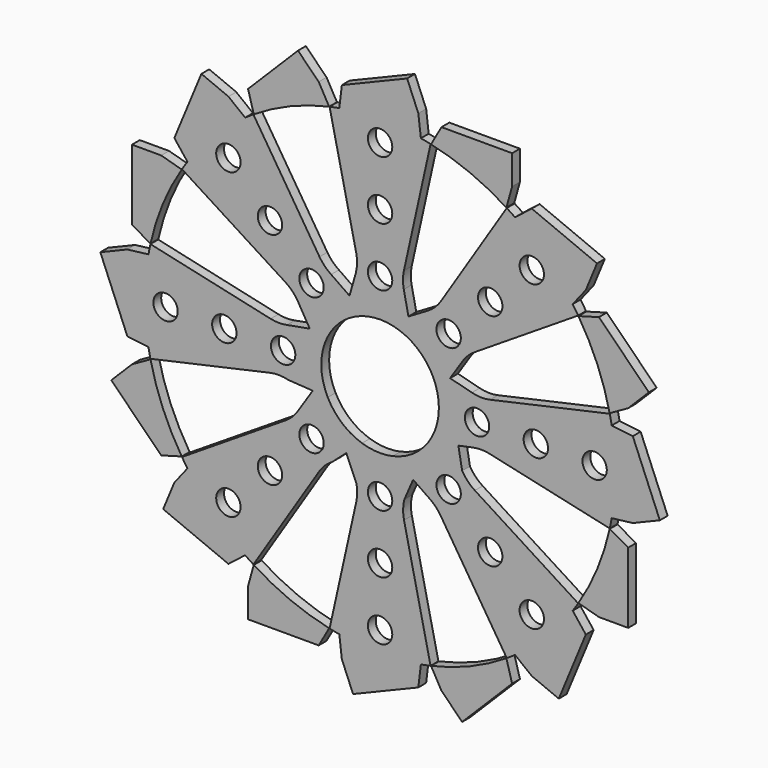
from build123d import *

# Parameters (mm, degrees)
F0_R     = 3.9501817168
F1_DEPTH = 3.175


# Not quite as in the source:
# - a feature names something its author has since deleted; it is built from what else it names


with BuildPart() as f1:
    # F0 (on Front) → F1 (new body)
    with BuildSketch(Plane.XZ):
        with BuildLine():
            ThreePointArc((-16.0654565205, 10.2373632733), (-10.9248771439, 15.6060744388), (-4.1210842565, 18.5989022405))
            Line((-4.1210842565, 18.5989022405), (-9.8997067311, 22.600704596))
            Line((-9.8997067311, 22.600704596), (-15.8721102734, 26.7367039053))
            ThreePointArc((-15.8721102734, 26.7367039053), (-17.9521481778, 28.4386641703), (-19.6274585749, 30.5402258516))
            Line((-19.6274585749, 30.5402258516), (-41.056319087, 64.1936029759))
            ThreePointArc((-41.056319087, 64.1936029759), (-42.3978695177, 63.3155641242), (-43.7206489599, 62.4094933045))
            ThreePointArc((-43.7206489599, 62.4094933045), (-53.8815367264, 53.8815367264), (-62.4094933045, 43.7206489599))
            ThreePointArc((-62.4094933045, 43.7206489599), (-63.3155641242, 42.3978695177), (-64.1936029759, 41.056319087))
            Line((-64.1936029759, 41.056319087), (-30.7105790862, 19.7359313647))
            ThreePointArc((-30.7105790862, 19.7359313647), (-28.3975370068, 17.8468155599), (-26.5895994967, 15.4697829255))
            Line((-26.5895994967, 15.4697829255), (-22.7875423577, 9.0161548324))
            Line((-22.7875423577, 9.0161548324), (-16.0654565205, 10.2373632733))
        make_face()
        with Locations((-22.2146216346, 22.2146216346)):
            Circle(F0_R, mode=Mode.SUBTRACT)
        with Locations((-35.6850058163, 35.6850058163)):
            Circle(F0_R, mode=Mode.SUBTRACT)
        with Locations((-49.1553899979, 49.1553899979)):
            Circle(F0_R, mode=Mode.SUBTRACT)
        with BuildLine():
            Line((30.5402258516, 19.6274585749), (64.1936029759, 41.056319087))
            ThreePointArc((64.1936029759, 41.056319087), (63.3155641242, 42.3978695177), (62.4094933045, 43.7206489599))
            ThreePointArc((62.4094933045, 43.7206489599), (53.8815367264, 53.8815367264), (43.7206489599, 62.4094933045))
            ThreePointArc((43.7206489599, 62.4094933045), (42.3978695177, 63.3155641242), (41.056319087, 64.1936029759))
            Line((41.056319087, 64.1936029759), (19.7359313647, 30.7105790862))
            ThreePointArc((19.7359313647, 30.7105790862), (17.8468155599, 28.3975370068), (15.4697829255, 26.5895994967))
            Line((15.4697829255, 26.5895994967), (9.1921845659, 22.8912476062))
            Line((9.1921845659, 22.8912476062), (7.682427832, 30.1289814441))
            ThreePointArc((7.682427832, 30.1289814441), (7.4150865693, 32.8032579961), (7.7164917428, 35.4739098544))
            Line((7.7164917428, 35.4739098544), (16.360530336, 74.42293361))
            ThreePointArc((16.360530336, 74.42293361), (14.791043703, 74.7506857907), (13.2150085686, 75.0453432835))
            ThreePointArc((13.2150085686, 75.0453432835), (0, 76.2), (-13.2150085686, 75.0453432835))
            ThreePointArc((-13.2150085686, 75.0453432835), (-14.791043703, 74.7506857907), (-16.360530336, 74.42293361))
            Line((-16.360530336, 74.42293361), (-7.760247825, 35.6710696271))
            ThreePointArc((-7.760247825, 35.6710696271), (-7.4604866815, 32.6996952915), (-7.8628977031, 29.7404745233))
            Line((-7.8628977031, 29.7404745233), (-9.8997067311, 22.600704596))
            Line((-9.8997067311, 22.600704596), (-4.1210842565, 18.5989022405))
            ThreePointArc((-4.1210842565, 18.5989022405), (6.4810916849, 17.913624719), (15.067414829, 11.6565651189))
            Line((15.067414829, 11.6565651189), (22.6864124527, 9.6867003717))
            Line((22.6864124527, 9.6867003717), (26.7367039053, 15.8721102734))
            ThreePointArc((26.7367039053, 15.8721102734), (28.4386641703, 17.9521481778), (30.5402258516, 19.6274585749))
        make_face()
        with Locations((22.2146216346, 22.2146216346)):
            Circle(F0_R, mode=Mode.SUBTRACT)
        with Locations((0, 31.4162191987)):
            Circle(F0_R, mode=Mode.SUBTRACT)
        with Locations((35.6850058163, 35.6850058163)):
            Circle(F0_R, mode=Mode.SUBTRACT)
        with Locations((0, 50.4662191987)):
            Circle(F0_R, mode=Mode.SUBTRACT)
        with Locations((0, 69.5162191987)):
            Circle(F0_R, mode=Mode.SUBTRACT)
        with Locations((49.1553899979, 49.1553899979)):
            Circle(F0_R, mode=Mode.SUBTRACT)
        with BuildLine():
            ThreePointArc((-16.9597401444, -8.6758120216), (-19.0287402006, 0.8997479525), (-16.0654565205, 10.2373632733))
            Line((-16.0654565205, 10.2373632733), (-22.7875423577, 9.0161548324))
            Line((-22.7875423577, 9.0161548324), (-30.1289814441, 7.682427832))
            ThreePointArc((-30.1289814441, 7.682427832), (-32.8032579961, 7.4150865693), (-35.4739098544, 7.7164917428))
            Line((-35.4739098544, 7.7164917428), (-74.42293361, 16.360530336))
            ThreePointArc((-74.42293361, 16.360530336), (-74.7506857907, 14.791043703), (-75.0453432835, 13.2150085686))
            ThreePointArc((-75.0453432835, 13.2150085686), (-76.2, 0), (-75.0453432835, -13.2150085686))
            ThreePointArc((-75.0453432835, -13.2150085686), (-74.7506857907, -14.791043703), (-74.42293361, -16.360530336))
            Line((-74.42293361, -16.360530336), (-35.6710696271, -7.760247825))
            ThreePointArc((-35.6710696271, -7.760247825), (-32.6996952915, -7.4604866815), (-29.7404745233, -7.8628977031))
            Line((-29.7404745233, -7.8628977031), (-21.8219612019, -8.3665520839))
            Line((-21.8219612019, -8.3665520839), (-16.9597401444, -8.6758120216))
        make_face()
        with Locations((-69.5162191987, 0)):
            Circle(F0_R, mode=Mode.SUBTRACT)
        with Locations((-50.4662191987, 0)):
            Circle(F0_R, mode=Mode.SUBTRACT)
        with Locations((-31.4162191987, 0)):
            Circle(F0_R, mode=Mode.SUBTRACT)
        with BuildLine():
            ThreePointArc((75.0453432835, -13.2150085686), (75.9107869746, -6.63267826), (76.2, 0))
            ThreePointArc((76.2, 0), (75.9107869746, 6.63267826), (75.0453432835, 13.2150085686))
            ThreePointArc((75.0453432835, 13.2150085686), (74.7506857907, 14.791043703), (74.42293361, 16.360530336))
            Line((74.42293361, 16.360530336), (35.6710696271, 7.760247825))
            ThreePointArc((35.6710696271, 7.760247825), (32.6996952915, 7.4604866815), (29.7404745233, 7.8628977031))
            Line((29.7404745233, 7.8628977031), (22.6864124527, 9.6867003717))
            Line((22.6864124527, 9.6867003717), (15.067414829, 11.6565651189))
            ThreePointArc((15.067414829, 11.6565651189), (18.0268792709, 6.1590684161), (19.05, 0))
            ThreePointArc((19.05, 0), (14.8561292921, -11.9246770379), (4.1210842565, -18.5989022405))
            Line((4.1210842565, -18.5989022405), (10.7153633273, -23.1655617921))
            Line((10.7153633273, -23.1655617921), (15.8721102734, -26.7367039053))
            ThreePointArc((15.8721102734, -26.7367039053), (17.9521481778, -28.4386641703), (19.6274585749, -30.5402258516))
            Line((19.6274585749, -30.5402258516), (41.056319087, -64.1936029759))
            ThreePointArc((41.056319087, -64.1936029759), (42.3978695177, -63.3155641242), (43.7206489599, -62.4094933045))
            ThreePointArc((43.7206489599, -62.4094933045), (53.8815367264, -53.8815367264), (62.4094933045, -43.7206489599))
            ThreePointArc((62.4094933045, -43.7206489599), (63.3155641242, -42.3978695177), (64.1936029759, -41.056319087))
            Line((64.1936029759, -41.056319087), (30.7105790862, -19.7359313647))
            ThreePointArc((30.7105790862, -19.7359313647), (28.3975370068, -17.8468155599), (26.5895994967, -15.4697829255))
            Line((26.5895994967, -15.4697829255), (25.3667239219, -8.6758120216))
            Line((25.3667239219, -8.6758120216), (30.1289814441, -7.682427832))
            ThreePointArc((30.1289814441, -7.682427832), (32.8032579961, -7.4150865693), (35.4739098544, -7.7164917428))
            Line((35.4739098544, -7.7164917428), (74.42293361, -16.360530336))
            ThreePointArc((74.42293361, -16.360530336), (74.7506857907, -14.791043703), (75.0453432835, -13.2150085686))
        make_face()
        with Locations((49.1553899979, -49.1553899979)):
            Circle(F0_R, mode=Mode.SUBTRACT)
        with Locations((35.6850058163, -35.6850058163)):
            Circle(F0_R, mode=Mode.SUBTRACT)
        with Locations((22.2146216346, -22.2146216346)):
            Circle(F0_R, mode=Mode.SUBTRACT)
        with Locations((31.4162191987, 0)):
            Circle(F0_R, mode=Mode.SUBTRACT)
        with Locations((50.4662191987, 0)):
            Circle(F0_R, mode=Mode.SUBTRACT)
        with Locations((69.5162191987, 0)):
            Circle(F0_R, mode=Mode.SUBTRACT)
        with BuildLine():
            Line((10.7153633273, -23.1655617921), (4.1210842565, -18.5989022405))
            ThreePointArc((4.1210842565, -18.5989022405), (-0.8997479525, -19.0287402006), (-5.8576217505, -18.127072776))
            Line((-5.8576217505, -18.127072776), (-10.9487517497, -22.609293046))
            Line((-10.9487517497, -22.609293046), (-7.682427832, -30.1289814441))
            ThreePointArc((-7.682427832, -30.1289814441), (-7.4150865693, -32.8032579961), (-7.7164917428, -35.4739098544))
            Line((-7.7164917428, -35.4739098544), (-16.360530336, -74.42293361))
            ThreePointArc((-16.360530336, -74.42293361), (-14.791043703, -74.7506857907), (-13.2150085686, -75.0453432835))
            ThreePointArc((-13.2150085686, -75.0453432835), (0, -76.2), (13.2150085686, -75.0453432835))
            ThreePointArc((13.2150085686, -75.0453432835), (14.791043703, -74.7506857907), (16.360530336, -74.42293361))
            Line((16.360530336, -74.42293361), (7.760247825, -35.6710696271))
            ThreePointArc((7.760247825, -35.6710696271), (7.4604866815, -32.6996952915), (7.8628977031, -29.7404745233))
            Line((7.8628977031, -29.7404745233), (10.7153633273, -23.1655617921))
        make_face()
        with Locations((0, -69.5162191987)):
            Circle(F0_R, mode=Mode.SUBTRACT)
        with Locations((0, -50.4662191987)):
            Circle(F0_R, mode=Mode.SUBTRACT)
        with Locations((0, -31.4162191987)):
            Circle(F0_R, mode=Mode.SUBTRACT)
        with BuildLine():
            Line((-10.9487517497, -22.609293046), (-5.8576217505, -18.127072776))
            ThreePointArc((-5.8576217505, -18.127072776), (-12.3486672732, -14.5056167251), (-16.9597401444, -8.6758120216))
            Line((-16.9597401444, -8.6758120216), (-21.8219612019, -8.3665520839))
            Line((-21.8219612019, -8.3665520839), (-26.7367039053, -15.8721102734))
            ThreePointArc((-26.7367039053, -15.8721102734), (-28.4386641703, -17.9521481778), (-30.5402258516, -19.6274585749))
            Line((-30.5402258516, -19.6274585749), (-64.1936029759, -41.056319087))
            ThreePointArc((-64.1936029759, -41.056319087), (-63.3155641242, -42.3978695177), (-62.4094933045, -43.7206489599))
            ThreePointArc((-62.4094933045, -43.7206489599), (-53.8815367264, -53.8815367264), (-43.7206489599, -62.4094933045))
            ThreePointArc((-43.7206489599, -62.4094933045), (-42.3978695177, -63.3155641242), (-41.056319087, -64.1936029759))
            Line((-41.056319087, -64.1936029759), (-19.7359313647, -30.7105790862))
            ThreePointArc((-19.7359313647, -30.7105790862), (-17.8468155599, -28.3975370068), (-15.4697829255, -26.5895994967))
            Line((-15.4697829255, -26.5895994967), (-10.9487517497, -22.609293046))
        make_face()
        with Locations((-49.1553899979, -49.1553899979)):
            Circle(F0_R, mode=Mode.SUBTRACT)
        with Locations((-35.6850058163, -35.6850058163)):
            Circle(F0_R, mode=Mode.SUBTRACT)
        with Locations((-22.2146216346, -22.2146216346)):
            Circle(F0_R, mode=Mode.SUBTRACT)
        with BuildLine():
            ThreePointArc((-75.0453432835, -13.2150085686), (-76.2, 0), (-75.0453432835, 13.2150085686))
            Line((-75.0453432835, 13.2150085686), (-81.8869620562, 12.3899634928))
            Line((-81.8869620562, 12.3899634928), (-90.6479892605, 8.7610272044))
            Line((-90.6479892605, 8.7610272044), (-81.8869620562, -12.3899634927))
            Line((-81.8869620562, -12.3899634927), (-75.0453432835, -13.2150085686))
        make_face()
        with BuildLine():
            ThreePointArc((-62.4094933045, 43.7206489599), (-53.8815367264, 53.8815367264), (-43.7206489599, 62.4094933045))
            Line((-43.7206489599, 62.4094933045), (-49.1417989563, 66.6638533651))
            Line((-49.1417989563, 66.6638533651), (-57.9028261607, 70.2927896534))
            Line((-57.9028261607, 70.2927896534), (-66.6638533651, 49.1417989563))
            Line((-66.6638533651, 49.1417989563), (-62.4094933045, 43.7206489599))
        make_face()
        with BuildLine():
            ThreePointArc((-13.2150085686, 75.0453432835), (0, 76.2), (13.2150085686, 75.0453432835))
            Line((13.2150085686, 75.0453432835), (12.3899634928, 81.8869620562))
            Line((12.3899634928, 81.8869620562), (8.7610272044, 90.6479892605))
            Line((8.7610272044, 90.6479892605), (-12.3899634927, 81.8869620562))
            Line((-12.3899634927, 81.8869620562), (-13.2150085686, 75.0453432835))
        make_face()
        with BuildLine():
            ThreePointArc((43.7206489599, 62.4094933045), (53.8815367264, 53.8815367264), (62.4094933045, 43.7206489599))
            Line((62.4094933045, 43.7206489599), (66.6638533651, 49.1417989563))
            Line((66.6638533651, 49.1417989563), (70.2927896534, 57.9028261607))
            Line((70.2927896534, 57.9028261607), (49.1417989563, 66.6638533651))
            Line((49.1417989563, 66.6638533651), (43.7206489599, 62.4094933045))
        make_face()
        with BuildLine():
            ThreePointArc((75.0453432835, 13.2150085686), (75.9107869746, 6.63267826), (76.2, 0))
            ThreePointArc((76.2, 0), (75.9107869746, -6.63267826), (75.0453432835, -13.2150085686))
            Line((75.0453432835, -13.2150085686), (81.8869620562, -12.3899634928))
            Line((81.8869620562, -12.3899634928), (90.6479892605, -8.7610272044))
            Line((90.6479892605, -8.7610272044), (81.8869620562, 12.3899634927))
            Line((81.8869620562, 12.3899634927), (75.0453432835, 13.2150085686))
        make_face()
        with BuildLine():
            Line((66.6638533651, -49.1417989563), (62.4094933045, -43.7206489599))
            ThreePointArc((62.4094933045, -43.7206489599), (53.8815367264, -53.8815367264), (43.7206489599, -62.4094933045))
            Line((43.7206489599, -62.4094933045), (49.1417989563, -66.6638533651))
            Line((49.1417989563, -66.6638533651), (57.9028261607, -70.2927896534))
            Line((57.9028261607, -70.2927896534), (66.6638533651, -49.1417989563))
        make_face()
        with BuildLine():
            Line((12.3899634927, -81.8869620562), (13.2150085686, -75.0453432835))
            ThreePointArc((13.2150085686, -75.0453432835), (0, -76.2), (-13.2150085686, -75.0453432835))
            Line((-13.2150085686, -75.0453432835), (-12.3899634928, -81.8869620562))
            Line((-12.3899634928, -81.8869620562), (-8.7610272044, -90.6479892605))
            Line((-8.7610272044, -90.6479892605), (12.3899634927, -81.8869620562))
        make_face()
        with BuildLine():
            Line((-49.1417989563, -66.6638533651), (-43.7206489599, -62.4094933045))
            ThreePointArc((-43.7206489599, -62.4094933045), (-53.8815367264, -53.8815367264), (-62.4094933045, -43.7206489599))
            Line((-62.4094933045, -43.7206489599), (-66.6638533651, -49.1417989563))
            Line((-66.6638533651, -49.1417989563), (-70.2927896534, -57.9028261607))
            Line((-70.2927896534, -57.9028261607), (-49.1417989563, -66.6638533651))
        make_face()
    extrude(amount=F1_DEPTH)


with BuildPart() as f1b:
    # F0 (on Front) → F1, piece 2 (new body)
    with BuildSketch(Plane.XZ):
        with BuildLine():
            Line((-80.3951219795, 19.8899500261), (-74.3900215076, 16.5095336123))
            ThreePointArc((-74.3900215076, 16.5095336123), (-70.3996203774, 29.1604775462), (-64.2756918321, 40.9276854892))
            Line((-64.2756918321, 40.9276854892), (-70.9122544669, 42.7836173851))
            Line((-70.9122544669, 42.7836173851), (-80.3951219795, 42.7836173851))
            Line((-80.3951219795, 42.7836173851), (-80.3951219795, 19.8899500261))
        make_face()
    extrude(amount=F1_DEPTH)


with BuildPart() as f1c:
    # F0 (on Front) → F1, piece 3 (new body)
    with BuildSketch(Plane.XZ):
        with BuildLine():
            Line((-42.7836173851, 70.9122544669), (-40.9276854892, 64.2756918321))
            ThreePointArc((-40.9276854892, 64.2756918321), (-29.1604775462, 70.3996203774), (-16.5095336123, 74.3900215076))
            Line((-16.5095336123, 74.3900215076), (-19.8899500261, 80.3951219795))
            Line((-19.8899500261, 80.3951219795), (-26.5953499493, 87.1005219027))
            Line((-26.5953499493, 87.1005219027), (-42.7836173851, 70.9122544669))
        make_face()
    extrude(amount=F1_DEPTH)


with BuildPart() as f1d:
    # F0 (on Front) → F1, piece 4 (new body)
    with BuildSketch(Plane.XZ):
        with BuildLine():
            ThreePointArc((16.5095336123, 74.3900215076), (29.1604775462, 70.3996203774), (40.9276854892, 64.2756918321))
            Line((40.9276854892, 64.2756918321), (42.7836173851, 70.9122544669))
            Line((42.7836173851, 70.9122544669), (42.7836173851, 80.3951219795))
            Line((42.7836173851, 80.3951219795), (19.8899500261, 80.3951219795))
            Line((19.8899500261, 80.3951219795), (16.5095336123, 74.3900215076))
        make_face()
    extrude(amount=F1_DEPTH)


with BuildPart() as f1e:
    # F0 (on Front) → F1, piece 5 (new body)
    with BuildSketch(Plane.XZ):
        with BuildLine():
            ThreePointArc((64.2756918321, 40.9276854892), (70.3996203774, 29.1604775462), (74.3900215076, 16.5095336123))
            Line((74.3900215076, 16.5095336123), (80.3951219795, 19.8899500261))
            Line((80.3951219795, 19.8899500261), (87.1005219027, 26.5953499493))
            Line((87.1005219027, 26.5953499493), (70.9122544669, 42.7836173851))
            Line((70.9122544669, 42.7836173851), (64.2756918321, 40.9276854892))
        make_face()
    extrude(amount=F1_DEPTH)


with BuildPart() as f1f:
    # F0 (on Front) → F1, piece 6 (new body)
    with BuildSketch(Plane.XZ):
        with BuildLine():
            Line((80.3951219795, -19.8899500261), (74.3900215076, -16.5095336123))
            ThreePointArc((74.3900215076, -16.5095336123), (70.3996203774, -29.1604775462), (64.2756918321, -40.9276854892))
            Line((64.2756918321, -40.9276854892), (70.9122544669, -42.7836173851))
            Line((70.9122544669, -42.7836173851), (80.3951219795, -42.7836173851))
            Line((80.3951219795, -42.7836173851), (80.3951219795, -19.8899500261))
        make_face()
    extrude(amount=F1_DEPTH)


with BuildPart() as f1g:
    # F0 (on Front) → F1, piece 7 (new body)
    with BuildSketch(Plane.XZ):
        with BuildLine():
            ThreePointArc((-64.2756918321, -40.9276854892), (-70.3996203774, -29.1604775462), (-74.3900215076, -16.5095336123))
            Line((-74.3900215076, -16.5095336123), (-80.3951219795, -19.8899500261))
            Line((-80.3951219795, -19.8899500261), (-87.1005219027, -26.5953499493))
            Line((-87.1005219027, -26.5953499493), (-70.9122544669, -42.7836173851))
            Line((-70.9122544669, -42.7836173851), (-64.2756918321, -40.9276854892))
        make_face()
    extrude(amount=F1_DEPTH)


with BuildPart() as f1h:
    # F0 (on Front) → F1, piece 8 (new body)
    with BuildSketch(Plane.XZ):
        with BuildLine():
            Line((42.7836173851, -70.9122544669), (40.9276854892, -64.2756918321))
            ThreePointArc((40.9276854892, -64.2756918321), (29.1604775462, -70.3996203774), (16.5095336123, -74.3900215076))
            Line((16.5095336123, -74.3900215076), (19.8899500261, -80.3951219795))
            Line((19.8899500261, -80.3951219795), (26.5953499493, -87.1005219027))
            Line((26.5953499493, -87.1005219027), (42.7836173851, -70.9122544669))
        make_face()
    extrude(amount=F1_DEPTH)


with BuildPart() as f1i:
    # F0 (on Front) → F1, piece 9 (new body)
    with BuildSketch(Plane.XZ):
        with BuildLine():
            ThreePointArc((-16.5095336123, -74.3900215076), (-29.1604775462, -70.3996203774), (-40.9276854892, -64.2756918321))
            Line((-40.9276854892, -64.2756918321), (-42.7836173851, -70.9122544669))
            Line((-42.7836173851, -70.9122544669), (-42.7836173851, -80.3951219795))
            Line((-42.7836173851, -80.3951219795), (-19.8899500261, -80.3951219795))
            Line((-19.8899500261, -80.3951219795), (-16.5095336123, -74.3900215076))
        make_face()
    extrude(amount=F1_DEPTH)


solid = Compound([f1.part, f1b.part, f1c.part, f1d.part, f1e.part, f1f.part, f1g.part, f1h.part, f1i.part])
